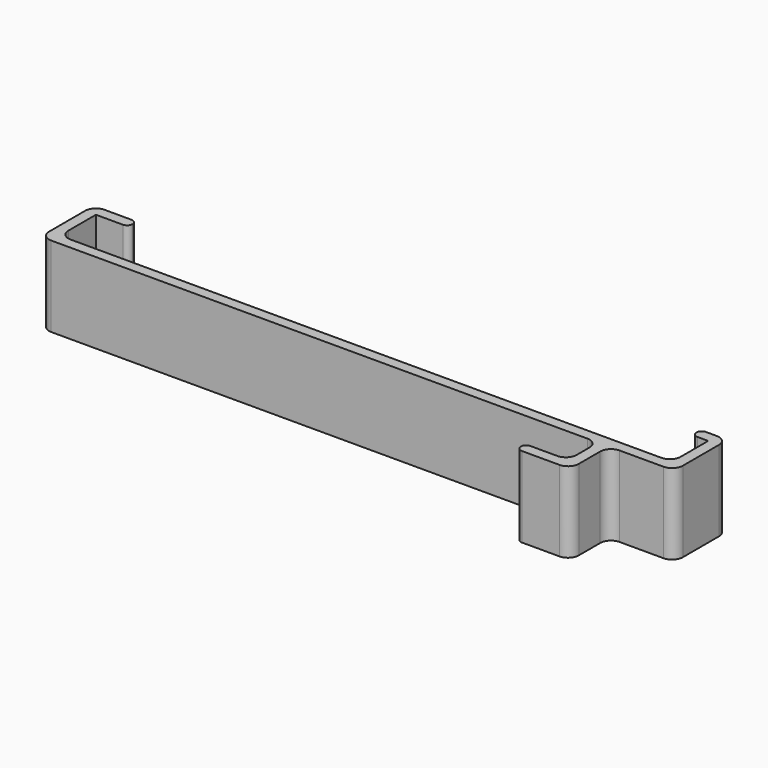
from build123d import *

# Parameters (mm, degrees)
F0_W     = 2
F0_H     = 7
F1_DEPTH = 15
F2_R     = 0.99999
F3_R     = 2


# Not quite as in the source:
# - a fillet or chamfer is up to 0.001 mm smaller than in the source, because OpenCascade refuses the exact size


with BuildPart() as f1:
    # F0 (on Top) → F1 (new body)
    with BuildSketch(Plane.XY):
        Polygon((61.5470979531, -0.0695097194), (-52.4529020469, -0.0695097194), (-52.4529020469, -2.0695097194), (49.3698753417, -2.0695097194), (51.3698753417, -2.0695097194), (61.5470979531, -2.0695097194), align=None)
        Polygon((-52.4529020469, -2.0695097194), (-52.4529020469, -0.0695097194), (-52.4529020469, 8.3304902806), (-54.4529020469, 8.3304902806), (-54.4529020469, -2.0695097194), align=None)
        Polygon((61.5470979531, 8.3304902806), (61.5470979531, -0.0695097194), (61.5470979531, -2.0695097194), (63.5470979531, -2.0695097194), (63.5470979531, 8.3304902806), align=None)
        Polygon((-54.4529020469, 8.3304902806), (-52.4529020469, 8.3304902806), (-46.4529020469, 8.3304902806), (-46.4529020469, 10.3304902806), (-54.4529020469, 10.3304902806), align=None)
        Polygon((58.5470979531, 8.3304902806), (61.5470979531, 8.3304902806), (63.5470979531, 8.3304902806), (63.5470979531, 10.3304902806), (58.5470979531, 10.3304902806), align=None)
        with Locations((50.3698753417, -5.5695097194)):
            Rectangle(F0_W, F0_H)
        Polygon((51.3698753417, -9.0695097194), (49.3698753417, -9.0695097194), (41.3698753417, -9.0695097194), (41.3698753417, -11.0695097194), (51.3698753417, -11.0695097194), align=None)
    extrude(amount=F1_DEPTH)

    # F2 (radius 1 in the source; OpenCascade refuses exactly that, so slightly less here)
    f2_edges = [f1.edges().sort_by_distance(p)[0] for p in [
        (58.547098, 10.33049, 7.5),
        (58.547098, 8.33049, 7.5),
        (-46.452902, 8.33049, 7.5),
        (-46.452902, 10.33049, 7.5),
        (41.369875, -9.06951, 7.5),
        (41.369875, -11.06951, 7.5),
    ]]
    fillet(f2_edges, radius=F2_R)

    # F3
    f3_edges = [f1.edges().sort_by_distance(p)[0] for p in [
        (-54.452902, 10.33049, 7.5),
        (-54.452902, -2.06951, 7.5),
        (63.547098, -2.06951, 7.5),
        (63.547098, 10.33049, 7.5),
        (51.369875, -11.06951, 7.5),
        (49.369875, -2.06951, 7.5),
        (51.369875, -2.06951, 7.5),
        (49.369875, -9.06951, 7.5),
        (-52.452902, -0.06951, 7.5),
        (61.547098, -0.06951, 7.5),
    ]]
    fillet(f3_edges, radius=F3_R)


solid = f1.part
